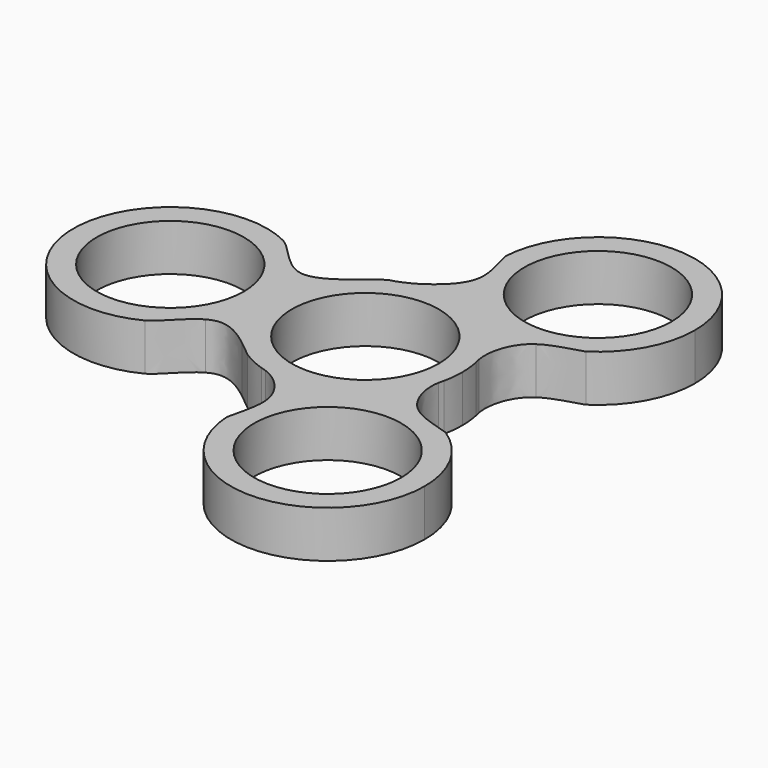
from build123d import *

# Parameters (mm, degrees)
F0_R     = 11
F1_DEPTH = 7


with BuildPart() as f1:
    # F0 (on Top) → F1 (new body)
    with BuildSketch(Plane.XY):
        with BuildLine():
            ThreePointArc((14.1759402298, -3.0483960701), (14.4187574592, -1.5327861344), (14.5, 0))
            ThreePointArc((14.5, 0), (14.421984404, 1.5021204517), (14.188777124, 2.9880769278))
            add(Edge.make_bspline(
                [(14.0117061641, 3.7312317498), (14.0561894605, 3.4787953407), (14.1150221965, 3.2304441785), (14.188777124, 2.9880769278)],
                knots=[0.9498383363, 0.9498383363, 0.9498383363, 0.9498383363, 1, 1, 1, 1], degree=3))
            ThreePointArc((14.0117061641, 3.7312317498), (7.1105429941, 12.6368579295), (-4.0835358776, 13.9131137685))
            add(Edge.make_bspline(
                [(-4.0835358776, 13.9131137685), (-4.9864056262, 13.4237848609), (-5.8861011392, 13.0613615019), (-6.6725668518, 12.8734941492)],
                knots=[0.8398981571, 0.8398981571, 0.8398981571, 0.8398981571, 1, 1, 1, 1], degree=3))
            ThreePointArc((-6.6725668518, 12.8734941492), (-7.25, 12.5573683549), (-7.8124895427, 12.2153594767))
            add(Edge.make_bspline(
                [(-10.3373118209, 10.1680865613), (-9.3752684105, 10.9198780403), (-8.503153556, 11.689001034), (-7.8124895427, 12.2153594767)],
                knots=[0.8153153807, 0.8153153807, 0.8153153807, 0.8153153807, 1, 1, 1, 1], degree=3))
            ThreePointArc((-10.3373118209, 10.1680865613), (-14.5, 0), (-10.3373118209, -10.1680865613))
            add(Edge.make_bspline(
                [(-10.3373118209, -10.1680865613), (-9.3752684105, -10.9198780403), (-8.503153556, -11.689001034), (-7.8124895427, -12.2153594767)],
                knots=[0.8153153807, 0.8153153807, 0.8153153807, 0.8153153807, 1, 1, 1, 1], degree=3))
            ThreePointArc((-7.8124895427, -12.2153594767), (-6.1812855522, -13.1164670899), (-4.4479816774, -13.8009223966))
            add(Edge.make_bspline(
                [(-3.7286645674, -14.0123895373), (-3.9647890084, -13.9271776533), (-4.2049522049, -13.8562123362), (-4.4479816774, -13.8009223966)],
                knots=[0.9507919436, 0.9507919436, 0.9507919436, 0.9507919436, 1, 1, 1, 1], degree=3))
            ThreePointArc((-3.7286645674, -14.0123895373), (7.25, -12.5573683549), (13.9994175907, -3.7770765311))
            add(Edge.make_bspline(
                [(13.9994175907, -3.7770765311), (14.043684155, -3.5299808247), (14.1023079859, -3.2865107369), (14.1759402298, -3.0483960701)],
                knots=[0.9507919436, 0.9507919436, 0.9507919436, 0.9507919436, 1, 1, 1, 1], degree=3))
        make_face()
        Circle(F0_R, mode=Mode.SUBTRACT)
        with BuildLine():
            ThreePointArc((-4.0835358776, 13.9131137685), (7.1105429941, 12.6368579295), (14.0117061641, 3.7312317498))
            add(Edge.make_bspline(
                [(16.8041360144, 10.9260038108), (16.4779875659, 10.7042997166), (14.5192375285, 9.1026767142), (13.6103052967, 6.0091248438), (14.0117061641, 3.7312317498)],
                knots=[0.4134483725, 0.4134483725, 0.4134483725, 0.4134483725, 0.4971979755, 0.9498383363, 0.9498383363, 0.9498383363, 0.9498383363], degree=3))
            ThreePointArc((16.8041360144, 10.9260038108), (7.4408037917, 12.6342244362), (1.1538261794, 19.7801267949))
            add(Edge.make_bspline(
                [(1.1538261794, 19.7801267949), (1.1027747103, 19.4661195397), (0.518142053, 17.2084365704), (-1.9632609294, 15.0622405677), (-4.0835358776, 13.9131137685)],
                knots=[0.4034852163, 0.4034852163, 0.4034852163, 0.4034852163, 0.4639193106, 0.8398981571, 0.8398981571, 0.8398981571, 0.8398981571], degree=3))
        make_face()
        with BuildLine():
            add(Edge.make_bspline(
                [(16.8324180589, -10.9304210804), (16.5090270331, -10.7103658028), (14.5525951809, -9.1161932679), (13.5913899182, -6.0546846446), (13.9994175907, -3.7770765311)],
                knots=[0.4137406454, 0.4137406454, 0.4137406454, 0.4137406454, 0.4972159985, 0.9507919436, 0.9507919436, 0.9507919436, 0.9507919436], degree=3))
            ThreePointArc((13.9994175907, -3.7770765311), (7.25, -12.5573683549), (-3.7286645674, -14.0123895373))
            add(Edge.make_bspline(
                [(1.0498133002, -20.0425121863), (1.0209353525, -19.6524197039), (0.6185573654, -17.1610137516), (-1.552184245, -14.7978312642), (-3.7286645674, -14.0123895373)],
                knots=[0.4137406454, 0.4137406454, 0.4137406454, 0.4137406454, 0.4972159985, 0.9507919436, 0.9507919436, 0.9507919436, 0.9507919436], degree=3))
            ThreePointArc((1.0498133002, -20.0425121863), (7.3307033346, -12.6971506308), (16.8324180589, -10.9304210804))
        make_face()
        with BuildLine():
            ThreePointArc((1.1538261794, 19.7801267949), (7.4408037917, 12.6342244362), (16.8041360144, 10.9260038108))
            add(Edge.make_bspline(
                [(22.4852798786, 13.0985463935), (20.5195105726, 12.423663188), (18.4142397082, 12.0204949315), (16.8041360144, 10.9260038108)],
                knots=[0, 0, 0, 0, 0.4134483725, 0.4134483725, 0.4134483725, 0.4134483725], degree=3))
            ThreePointArc((22.4852798786, 13.0985463935), (27.3256309509, 18.3395482658), (29.0807033346, 25.2545189857))
            ThreePointArc((29.0807033346, 25.2545189857), (14.964626833, 39.7494354307), (0.1010339902, 26.0220967828))
            add(Edge.make_bspline(
                [(0.1010339902, 26.0220967828), (0.5023641828, 24.0338894608), (1.4946687664, 21.8765805705), (1.1538261794, 19.7801267949)],
                knots=[0, 0, 0, 0, 0.4034852163, 0.4034852163, 0.4034852163, 0.4034852163], degree=3))
        make_face()
        with Locations((14.5807033346, 25.2545189857)):
            Circle(F0_R, mode=Mode.SUBTRACT)
        with BuildLine():
            add(Edge.make_bspline(
                [(22.4852798786, -13.0985463935), (20.5122225081, -12.4305468552), (18.4352865313, -12.0211120353), (16.8324180589, -10.9304210804)],
                knots=[0, 0, 0, 0, 0.4137406454, 0.4137406454, 0.4137406454, 0.4137406454], degree=3))
            ThreePointArc((16.8324180589, -10.9304210804), (7.3307033346, -12.6971506308), (1.0498133002, -20.0425121863))
            add(Edge.make_bspline(
                [(0.1010339902, -26.0220967828), (0.5090581055, -23.9793792077), (1.1929451387, -21.9759824798), (1.0498133002, -20.0425121863)],
                knots=[0, 0, 0, 0, 0.4137406454, 0.4137406454, 0.4137406454, 0.4137406454], degree=3))
            ThreePointArc((0.1010339902, -26.0220967828), (14.964626833, -39.7494354307), (29.0807033346, -25.2545189857))
            ThreePointArc((29.0807033346, -25.2545189857), (27.3256309509, -18.3395482658), (22.4852798786, -13.0985463935))
        make_face()
        with Locations((14.5807033346, -25.2545189857)):
            Circle(F0_R, mode=Mode.SUBTRACT)
        with BuildLine():
            ThreePointArc((-10.3373118209, -10.1680865613), (-14.5, 0), (-10.3373118209, 10.1680865613))
            add(Edge.make_bspline(
                [(-17.2748335615, 8.3041784514), (-16.7684606801, 8.0190428188), (-14.5727828059, 7.2074422158), (-12.0132482268, 8.8584214299), (-10.3373118209, 10.1680865613)],
                knots=[0.3927670048, 0.3927670048, 0.3927670048, 0.3927670048, 0.4935838728, 0.8153153807, 0.8153153807, 0.8153153807, 0.8153153807], degree=3))
            ThreePointArc((-17.2748335615, 8.3041784514), (-15.3301863677, 4.3528548067), (-14.6614066693, 0))
            ThreePointArc((-14.6614066693, 0), (-15.3301863677, -4.3528548067), (-17.2748335615, -8.3041784514))
            add(Edge.make_bspline(
                [(-17.2748335615, -8.3041784514), (-16.7684606801, -8.0190428188), (-14.5727828059, -7.2074422158), (-12.0132482268, -8.8584214299), (-10.3373118209, -10.1680865613)],
                knots=[0.3927670048, 0.3927670048, 0.3927670048, 0.3927670048, 0.4935838728, 0.8153153807, 0.8153153807, 0.8153153807, 0.8153153807], degree=3))
        make_face()
        with BuildLine():
            ThreePointArc((-14.6614066693, 0), (-15.3301863677, 4.3528548067), (-17.2748335615, 8.3041784514))
            add(Edge.make_bspline(
                [(-22.5863138688, 12.9235503893), (-20.9547365723, 11.9145258046), (-19.2475843898, 9.4150230013), (-17.2748335615, 8.3041784514)],
                knots=[0, 0, 0, 0, 0.3927670048, 0.3927670048, 0.3927670048, 0.3927670048], degree=3))
            ThreePointArc((-22.5863138688, 12.9235503893), (-43.6614066693, 0), (-22.5863138688, -12.9235503893))
            add(Edge.make_bspline(
                [(-22.5863138688, -12.9235503893), (-20.9547365723, -11.9145258046), (-19.2475843898, -9.4150230013), (-17.2748335615, -8.3041784514)],
                knots=[0, 0, 0, 0, 0.3927670048, 0.3927670048, 0.3927670048, 0.3927670048], degree=3))
            ThreePointArc((-17.2748335615, -8.3041784514), (-15.3301863677, -4.3528548067), (-14.6614066693, 0))
        make_face()
        with Locations((-29.1614066693, 0)):
            Circle(F0_R, mode=Mode.SUBTRACT)
    extrude(amount=F1_DEPTH)


solid = f1.part
